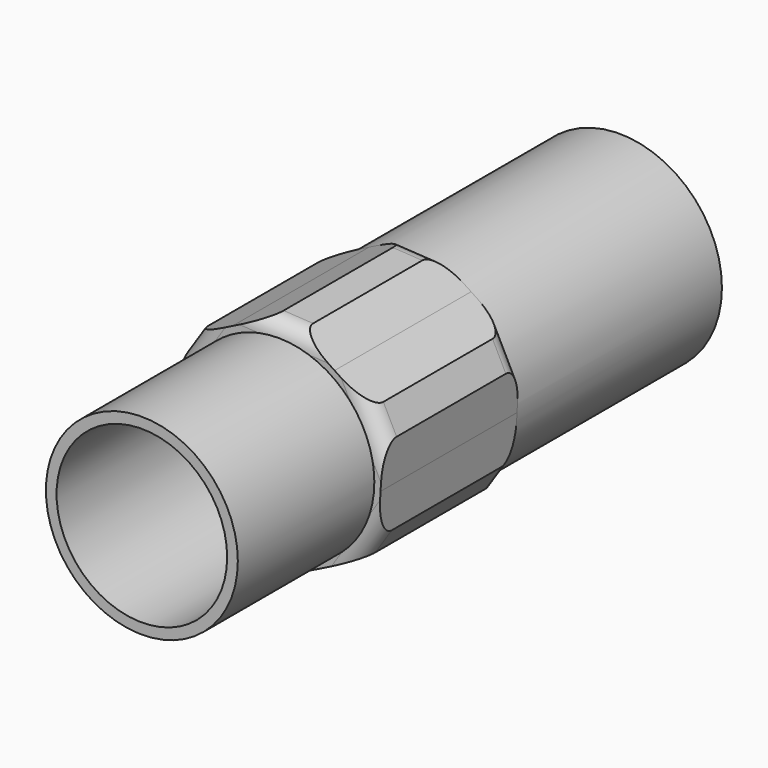
from build123d import *

# Parameters (mm, degrees)
F0_R         = 7.62
F1_DEPTH     = 19.05
F3_DEPTH     = 12.7
F4_SIZE      = 1.27
F5_T1_DEPTH  = 8.5497045256
F5_T3_DEPTH  = 8.5497045256
F5_T5_DEPTH  = 8.5497045256
F5_T7_DEPTH  = 8.5497045256
F5_T12_DEPTH = 8.5497045256
F5_S13_R     = 7.62
F5_T14_DEPTH = 6
F5_T18_DEPTH = 8.5497045256
F5_S19_R     = 7.62
F5_T20_DEPTH = 6
F5_T24_DEPTH = 8.5497045256
F5_S25_R     = 7.62
F5_T26_DEPTH = 6
F5_T30_DEPTH = 8.5497045256
F5_S31_R     = 7.62
F5_T32_DEPTH = 6
F5_T36_DEPTH = 8.5497045256
F5_S37_R     = 7.62
F5_T38_DEPTH = 6
F5_T42_DEPTH = 8.5497045256
F5_S43_R     = 7.62
F5_T44_DEPTH = 6
F6_R         = 7.14375
F7_DEPTH     = 12.7
F8_R         = 6.35
F9_DEPTH     = 44.4510001


# Not quite as in the source:
# - a fillet or chamfer that OpenCascade refuses, or shapes differently, is made with other operations: its cross-section is extruded or revolved along the edge and cut away or added


with BuildPart() as f1:
    # F0 (on Front) → F1 (new body)
    with BuildSketch(Plane.XZ):
        Circle(F0_R)
    extrude(amount=F1_DEPTH)

    # F2 (on face) → F3 (join)
    with BuildSketch(Plane.XZ.offset(19.05)):
        with BuildLine():
            Line((7.8629215405, 3.9488814679), (4.1872753391, 6.3664059904))
            ThreePointArc((4.1872753391, 6.3664059904), (6.7071394083, 3.6164459015), (7.62, 0))
            ThreePointArc((7.62, 0), (7.616776064, -0.2216357159), (7.6071069841, -0.4430838887))
            Line((7.6071069841, -0.4430838887), (7.8629215405, 3.9488814679))
        make_face()
        with BuildLine():
            ThreePointArc((4.1872753391, 6.3664059904), (0.4430838236, 7.6071069879), (-3.4198316443, 6.8094898138))
            ThreePointArc((-3.4198316443, 6.8094898138), (-6.3664059346, 4.187275424), (-7.6071069765, 0.4430840189))
            ThreePointArc((-7.6071069765, 0.4430840189), (-6.8094898664, -3.4198315396), (-4.187275378, -6.3664059648))
            ThreePointArc((-4.187275378, -6.3664059648), (-0.4430838337, -7.6071069873), (3.419831668, -6.8094898019))
            ThreePointArc((3.419831668, -6.8094898019), (6.3664059777, -4.1872753585), (7.6071069841, -0.4430838887))
            ThreePointArc((7.6071069841, -0.4430838887), (7.616776064, -0.2216357159), (7.62, 0))
            ThreePointArc((7.62, 0), (6.7071394083, 3.6164459015), (4.1872753391, 6.3664059904))
        make_face()
        with BuildLine():
            ThreePointArc((7.6071069841, -0.4430838887), (6.3664059777, -4.1872753585), (3.419831668, -6.8094898019))
            Line((3.419831668, -6.8094898019), (7.351292438, -4.8350490681))
            Line((7.351292438, -4.8350490681), (7.6071069841, -0.4430838887))
        make_face()
        with BuildLine():
            ThreePointArc((3.419831668, -6.8094898019), (-0.4430838337, -7.6071069873), (-4.187275378, -6.3664059648))
            Line((-4.187275378, -6.3664059648), (-0.5116291025, -8.783930536))
            Line((-0.5116291025, -8.783930536), (3.419831668, -6.8094898019))
        make_face()
        with BuildLine():
            ThreePointArc((-4.187275378, -6.3664059648), (-6.8094898664, -3.4198315396), (-7.6071069765, 0.4430840189))
            Line((-7.6071069765, 0.4430840189), (-7.8629215405, -3.9488814679))
            Line((-7.8629215405, -3.9488814679), (-4.187275378, -6.3664059648))
        make_face()
        with BuildLine():
            Line((-3.4198316443, 6.8094898138), (-7.351292438, 4.8350490681))
            Line((-7.351292438, 4.8350490681), (-7.6071069765, 0.4430840189))
            ThreePointArc((-7.6071069765, 0.4430840189), (-6.3664059346, 4.187275424), (-3.4198316443, 6.8094898138))
        make_face()
        with BuildLine():
            Line((0.5116291025, 8.783930536), (-3.4198316443, 6.8094898138))
            ThreePointArc((-3.4198316443, 6.8094898138), (0.4430838236, 7.6071069879), (4.1872753391, 6.3664059904))
            Line((4.1872753391, 6.3664059904), (0.5116291025, 8.783930536))
        make_face()
    extrude(amount=F3_DEPTH)

    # F4
    f4_edges = [f1.edges().sort_by_distance(p)[0] for p in [
        (7.862922, -25.4, 3.948881),
        (7.351292, -25.4, -4.835049),
        (-0.511629, -25.4, -8.783931),
        (-7.862922, -25.4, -3.948881),
        (-7.351292, -25.4, 4.835049),
        (0.511629, -25.4, 8.783931),
    ]]
    chamfer(f4_edges, length=F4_SIZE)

    # F5: fillet of radius 1.27 on 12 edges, made by hand

    # F5_s2 → F5_t1 (cut)
    with BuildSketch(Plane(origin=(1.918540045, 0, -3.8201526101), x_dir=(0, 1, 0), z_dir=(-0.4487968068, 0, 0.8936338323))):
        with BuildLine():
            ThreePointArc((-30.48, -8.1638181024), (-31.3780256121, -7.7918437146), (-31.75, -6.8938181024))
            Line((-31.75, -6.8938181024), (-31.75, -8.1638181024))
            Line((-31.75, -8.1638181024), (-30.48, -8.1638181024))
        make_face()
        with BuildLine():
            ThreePointArc((-31.75, 6.8938181024), (-31.3780256121, 7.7918437146), (-30.48, 8.1638181024))
            Line((-30.48, 8.1638181024), (-31.75, 8.1638181024))
            Line((-31.75, 8.1638181024), (-31.75, 6.8938181024))
        make_face()
    extrude(amount=F5_T1_DEPTH, mode=Mode.SUBTRACT)

    # F5_s4 → F5_t3 (cut)
    with BuildSketch(Plane(origin=(4.2676192292, 0, -0.2485718879), x_dir=(0, 1, 0), z_dir=(-0.9983080038, 0, 0.0581474803))):
        with BuildLine():
            ThreePointArc((-31.75, -6.8938181024), (-31.3780256121, -7.7918437146), (-30.48, -8.1638181024))
            Line((-30.48, -8.1638181024), (-31.75, -8.1638181024))
            Line((-31.75, -8.1638181024), (-31.75, -6.8938181024))
        make_face()
        with BuildLine():
            ThreePointArc((-31.75, 6.8938181024), (-31.3780256121, 7.7918437146), (-30.48, 8.1638181024))
            Line((-30.48, 8.1638181024), (-31.75, 8.1638181024))
            Line((-31.75, 8.1638181024), (-31.75, 6.8938181024))
        make_face()
    extrude(amount=F5_T3_DEPTH, mode=Mode.SUBTRACT)

    # F5_s6 → F5_t5 (cut)
    with BuildSketch(Plane(origin=(-2.3490791841, 0, -3.5715807222), x_dir=(0, 1, 0), z_dir=(0.5495111971, 0, 0.835486352))):
        with BuildLine():
            ThreePointArc((-31.75, 6.8938181024), (-31.3780256121, 7.7918437146), (-30.48, 8.1638181024))
            Line((-30.48, 8.1638181024), (-31.75, 8.1638181024))
            Line((-31.75, 8.1638181024), (-31.75, 6.8938181024))
        make_face()
    extrude(amount=F5_T5_DEPTH, mode=Mode.SUBTRACT)

    # F5_s8 → F5_t7 (cut)
    with BuildSketch(Plane(origin=(2.3490791841, 0, 3.5715807222), x_dir=(0, 1, 0), z_dir=(-0.5495111971, 0, -0.835486352))):
        with BuildLine():
            ThreePointArc((-30.48, 8.1638181024), (-31.3780256121, 7.7918437146), (-31.75, 6.8938181024))
            Line((-31.75, 6.8938181024), (-31.75, 8.1638181024))
            Line((-31.75, 8.1638181024), (-30.48, 8.1638181024))
        make_face()
    extrude(amount=F5_T7_DEPTH, mode=Mode.SUBTRACT)


with BuildPart() as f5_tool10:
    # F5_s11 → F5_t12 (new body)
    with BuildSketch(Plane(origin=(4.2676192292, 0, -0.2485718879), x_dir=(0, 1, 0), z_dir=(-0.9983080038, 0, 0.0581474803))):
        with BuildLine():
            ThreePointArc((-19.05, -6.8938181024), (-19.4219743879, -7.7918437146), (-20.32, -8.1638181024))
            Line((-20.32, -8.1638181024), (-19.05, -8.1638181024))
            Line((-19.05, -8.1638181024), (-19.05, -6.8938181024))
        make_face()
    extrude(amount=F5_T12_DEPTH)

    # F5_s13 → F5_t14 (cut, symmetric)
    with BuildSketch(Plane.XZ.offset(19.7)):
        Circle(F5_S13_R)
    extrude(amount=F5_T14_DEPTH, both=True, mode=Mode.SUBTRACT)


with BuildPart() as f1_1:
    add(f1.part)

    # F5_t9: cut F5_tool10
    add(f5_tool10.part, mode=Mode.SUBTRACT)


with BuildPart() as f5_tool16:
    # F5_s17 → F5_t18 (new body)
    with BuildSketch(Plane(origin=(-2.3490791841, 0, -3.5715807222), x_dir=(0, 1, 0), z_dir=(0.5495111971, 0, 0.835486352))):
        with BuildLine():
            ThreePointArc((-19.05, 6.8938181024), (-19.4219743879, 7.7918437146), (-20.32, 8.1638181024))
            Line((-20.32, 8.1638181024), (-19.05, 8.1638181024))
            Line((-19.05, 8.1638181024), (-19.05, 6.8938181024))
        make_face()
    extrude(amount=F5_T18_DEPTH)

    # F5_s19 → F5_t20 (cut, symmetric)
    with BuildSketch(Plane.XZ.offset(19.7)):
        Circle(F5_S19_R)
    extrude(amount=F5_T20_DEPTH, both=True, mode=Mode.SUBTRACT)


with BuildPart() as f1_2:
    add(f1_1.part)

    # F5_t15: cut F5_tool16
    add(f5_tool16.part, mode=Mode.SUBTRACT)


with BuildPart() as f5_tool22:
    # F5_s23 → F5_t24 (new body)
    with BuildSketch(Plane(origin=(1.918540045, 0, -3.8201526101), x_dir=(0, 1, 0), z_dir=(-0.4487968068, 0, 0.8936338323))):
        with BuildLine():
            ThreePointArc((-19.05, 6.8938181024), (-19.4219743879, 7.7918437146), (-20.32, 8.1638181024))
            Line((-20.32, 8.1638181024), (-19.05, 8.1638181024))
            Line((-19.05, 8.1638181024), (-19.05, 6.8938181024))
        make_face()
    extrude(amount=F5_T24_DEPTH)

    # F5_s25 → F5_t26 (cut, symmetric)
    with BuildSketch(Plane.XZ.offset(19.7)):
        Circle(F5_S25_R)
    extrude(amount=F5_T26_DEPTH, both=True, mode=Mode.SUBTRACT)


with BuildPart() as f1_3:
    add(f1_2.part)

    # F5_t21: cut F5_tool22
    add(f5_tool22.part, mode=Mode.SUBTRACT)


with BuildPart() as f5_tool28:
    # F5_s29 → F5_t30 (new body)
    with BuildSketch(Plane(origin=(4.2676192292, 0, -0.2485718879), x_dir=(0, 1, 0), z_dir=(-0.9983080038, 0, 0.0581474803))):
        with BuildLine():
            ThreePointArc((-19.05, 6.8938181024), (-19.4219743879, 7.7918437146), (-20.32, 8.1638181024))
            Line((-20.32, 8.1638181024), (-19.05, 8.1638181024))
            Line((-19.05, 8.1638181024), (-19.05, 6.8938181024))
        make_face()
    extrude(amount=F5_T30_DEPTH)

    # F5_s31 → F5_t32 (cut, symmetric)
    with BuildSketch(Plane.XZ.offset(19.7)):
        Circle(F5_S31_R)
    extrude(amount=F5_T32_DEPTH, both=True, mode=Mode.SUBTRACT)


with BuildPart() as f1_4:
    add(f1_3.part)

    # F5_t27: cut F5_tool28
    add(f5_tool28.part, mode=Mode.SUBTRACT)


with BuildPart() as f5_tool34:
    # F5_s35 → F5_t36 (new body)
    with BuildSketch(Plane(origin=(2.3490791841, 0, 3.5715807222), x_dir=(0, 1, 0), z_dir=(-0.5495111971, 0, -0.835486352))):
        with BuildLine():
            ThreePointArc((-19.05, 6.8938181024), (-19.4219743879, 7.7918437146), (-20.32, 8.1638181024))
            Line((-20.32, 8.1638181024), (-19.05, 8.1638181024))
            Line((-19.05, 8.1638181024), (-19.05, 6.8938181024))
        make_face()
    extrude(amount=F5_T36_DEPTH)

    # F5_s37 → F5_t38 (cut, symmetric)
    with BuildSketch(Plane.XZ.offset(19.7)):
        Circle(F5_S37_R)
    extrude(amount=F5_T38_DEPTH, both=True, mode=Mode.SUBTRACT)


with BuildPart() as f1_5:
    add(f1_4.part)

    # F5_t33: cut F5_tool34
    add(f5_tool34.part, mode=Mode.SUBTRACT)


with BuildPart() as f5_tool40:
    # F5_s41 → F5_t42 (new body)
    with BuildSketch(Plane(origin=(1.918540045, 0, -3.8201526101), x_dir=(0, 1, 0), z_dir=(-0.4487968068, 0, 0.8936338323))):
        with BuildLine():
            ThreePointArc((-19.05, -6.8938181024), (-19.4219743879, -7.7918437146), (-20.32, -8.1638181024))
            Line((-20.32, -8.1638181024), (-19.05, -8.1638181024))
            Line((-19.05, -8.1638181024), (-19.05, -6.8938181024))
        make_face()
    extrude(amount=F5_T42_DEPTH)

    # F5_s43 → F5_t44 (cut, symmetric)
    with BuildSketch(Plane.XZ.offset(19.7)):
        Circle(F5_S43_R)
    extrude(amount=F5_T44_DEPTH, both=True, mode=Mode.SUBTRACT)


with BuildPart() as f1_6:
    add(f1_5.part)

    # F5_t39: cut F5_tool40
    add(f5_tool40.part, mode=Mode.SUBTRACT)

    # F6 (on face) → F7 (join)
    with BuildSketch(Plane.XZ.offset(31.75)):
        Circle(F6_R)
    extrude(amount=F7_DEPTH)

    # F8 (on face) → F9 (cut, through all)
    with BuildSketch(Plane.XZ.offset(44.45)):
        Circle(F8_R)
    extrude(amount=-F9_DEPTH, mode=Mode.SUBTRACT)


solid = f1_6.part
